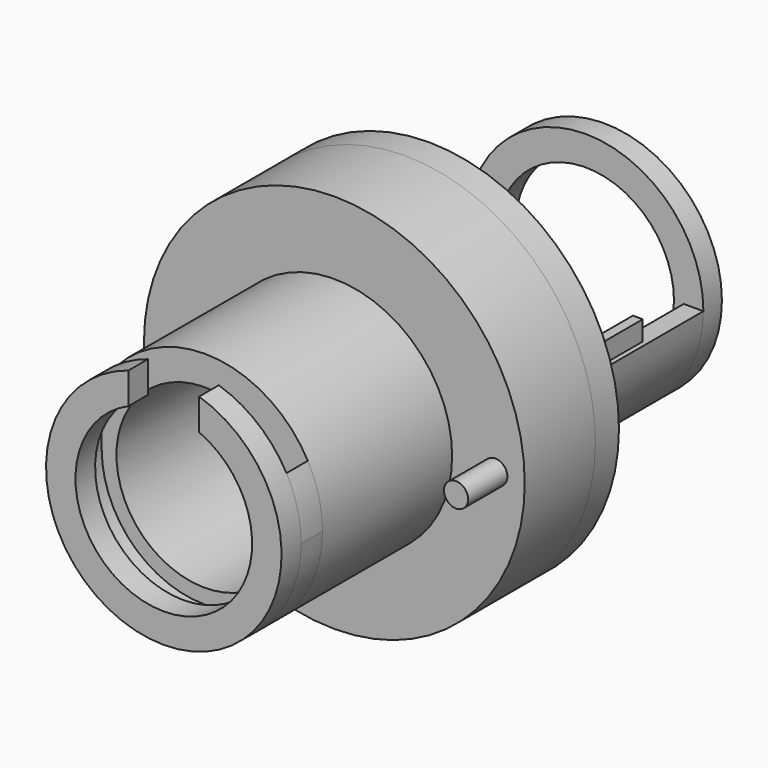
from build123d import *

# Parameters (mm, degrees)
F0_R      = 15.24
F0_R_2    = 11.43
F1_DEPTH  = 2.9972
F3_DEPTH  = 26.67
F4_R      = 15.24
F4_R_2    = 11.43
F5_DEPTH  = 2.54
F6_W      = 9.144
F6_H      = 6.35
F7_DEPTH  = 28.575
F8_W      = 1.27
F8_H      = 6.096
F9_DEPTH  = 2.54
F10_R     = 24.638
F10_R_2   = 15.24
F11_DEPTH = 3.81
F12_DEPTH = 11.43
F13_R     = 15.24
F13_R_2   = 11.43
F14_DEPTH = 20.955
F16_DEPTH = 3.4544
F17_R     = 15.24
F17_R_2   = 11.43
F18_DEPTH = 3.175
F19_DEPTH = 25.4
F20_R     = 1.5621
F21_DEPTH = 6.35


with BuildPart() as f1:
    # F0 (on Front) → F1 (new body)
    with BuildSketch(Plane.XZ):
        Circle(F0_R)
        Circle(F0_R_2, mode=Mode.SUBTRACT)
    extrude(amount=F1_DEPTH)

    # F2 (on face) → F3 (join)
    with BuildSketch(Plane.XZ.offset(2.9972)):
        with BuildLine():
            Line((15.24, 0), (12.7, 0))
            ThreePointArc((12.7, 0), (0, -12.7), (-12.7, 0))
            Line((-12.7, 0), (-15.24, 0))
            ThreePointArc((-15.24, 0), (0, -15.24), (15.24, 0))
        make_face()
    extrude(amount=F3_DEPTH)

    # F4 (on face) → F5 (join)
    with BuildSketch(Plane.XZ.offset(29.6672)):
        Circle(F4_R)
        Circle(F4_R_2, mode=Mode.SUBTRACT)
    extrude(amount=F5_DEPTH)

    # F6 (on Top) → F7 (cut)
    with BuildSketch(Plane.XY):
        Polygon((-13.335, -64.7192), (-13.335, -68.0212), (-4.572, -68.0212), (4.572, -68.0212), (13.335, -68.0212), (13.335, -64.7192), align=None)
        with Locations((0, -71.1962)):
            Rectangle(F6_W, F6_H)
    extrude(amount=F7_DEPTH, mode=Mode.SUBTRACT)

    # F8 (on face) → F9 (join)
    with BuildSketch(Plane.XY):
        with Locations((13.97, -15.0622)):
            Rectangle(F8_W, F8_H)
        with Locations((-13.97, -15.0622)):
            Rectangle(F8_W, F8_H)
    extrude(amount=F9_DEPTH)

    # F10 (on face) → F11 (join)
    with BuildSketch(Plane.XZ.offset(32.2072)):
        Circle(F10_R)
        Circle(F10_R_2, mode=Mode.SUBTRACT)
    extrude(amount=-F11_DEPTH)

    # F12 (add): a face of the model
    f12_faces = [f1.faces().sort_by_distance(p)[0] for p in [
        (-23.941132125, -32.2072, 0),
    ]]
    extrude(f12_faces, amount=F12_DEPTH)

    # F13 (on face) → F14 (join)
    with BuildSketch(Plane.XZ.offset(43.6372)):
        Circle(F13_R)
        Circle(F13_R_2, mode=Mode.SUBTRACT)
    extrude(amount=F14_DEPTH)

    # F15 (on face) → F16 (join)
    with BuildSketch(Plane.XZ.offset(64.5922)):
        with BuildLine():
            Line((13.335, 7.3780332745), (13.335, 0))
            ThreePointArc((13.335, 0), (0, -13.335), (-13.335, 0))
            Line((-13.335, 0), (-13.335, 7.3780332745))
            ThreePointArc((-13.335, 7.3780332745), (-3.81, -14.7560665491), (15.24, 0))
            ThreePointArc((15.24, 0), (14.7560665491, 3.81), (13.335, 7.3780332745))
        make_face()
    extrude(amount=F16_DEPTH)

    # F17 (on face) → F18 (join)
    with BuildSketch(Plane.XZ.offset(68.0466)):
        Circle(F17_R)
        Circle(F17_R_2, mode=Mode.SUBTRACT)
    extrude(amount=F18_DEPTH)

    # F6 (on Top) → F19 (cut)
    with BuildSketch(Plane.XY):
        Polygon((-13.335, -64.7192), (-13.335, -68.0212), (-4.572, -68.0212), (4.572, -68.0212), (13.335, -68.0212), (13.335, -64.7192), align=None)
        with Locations((0, -71.1962)):
            Rectangle(F6_W, F6_H)
    extrude(amount=F19_DEPTH, mode=Mode.SUBTRACT)

    # F20 (on face) → F21 (join)
    with BuildSketch(Plane.XZ.offset(43.6372)):
        with Locations((20.828, 0)):
            Circle(F20_R)
        with Locations((-20.828, 0)):
            Circle(F20_R)
    extrude(amount=F21_DEPTH)


solid = f1.part
